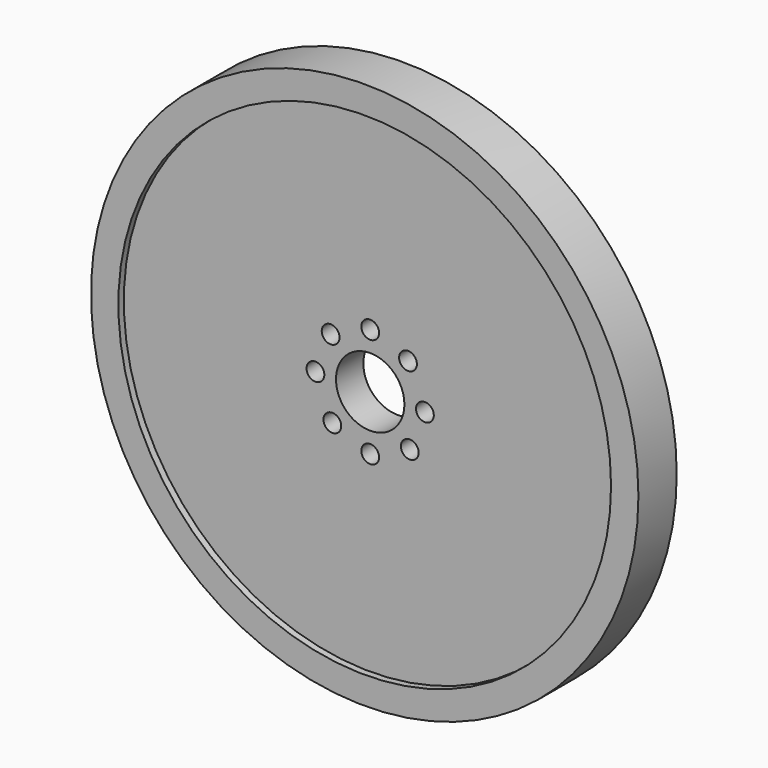
from build123d import *

# Parameters (mm, degrees)
F0_R     = 50.8
F0_R_2   = 45.72
F1_DEPTH = 4.445
F0_R_3   = 6.35
F2_DEPTH = 3.175
F4_D     = 3.3


# Not quite as in the source:
# - a feature names something its author has since deleted; it is built from what else it names


with BuildPart() as f1:
    # F0 (on Front) → F1 (new body, symmetric)
    with BuildSketch(Plane.XZ):
        Circle(F0_R)
        Circle(F0_R_2, mode=Mode.SUBTRACT)
    extrude(amount=F1_DEPTH, both=True)


with BuildPart() as f2:
    # F0 (on Front) → F2 (new body, symmetric)
    with BuildSketch(Plane.XZ):
        Circle(F0_R_2)
        Circle(F0_R_3, mode=Mode.SUBTRACT)
    extrude(amount=F2_DEPTH, both=True)

    # F4 (through all)
    with Locations(Plane.XZ.offset(3.175)):
        with Locations((10.16, 0), (7.3437980366, -7.0209850019), (0, -10.16), (-7.0209850019, -7.3437980366), (-10.16, 0), (-7.3437980366, 7.0209850019), (0, 10.16), (7.0209850019, 7.3437980366)):
            Hole(F4_D / 2)


solid = Compound([f1.part, f2.part])
